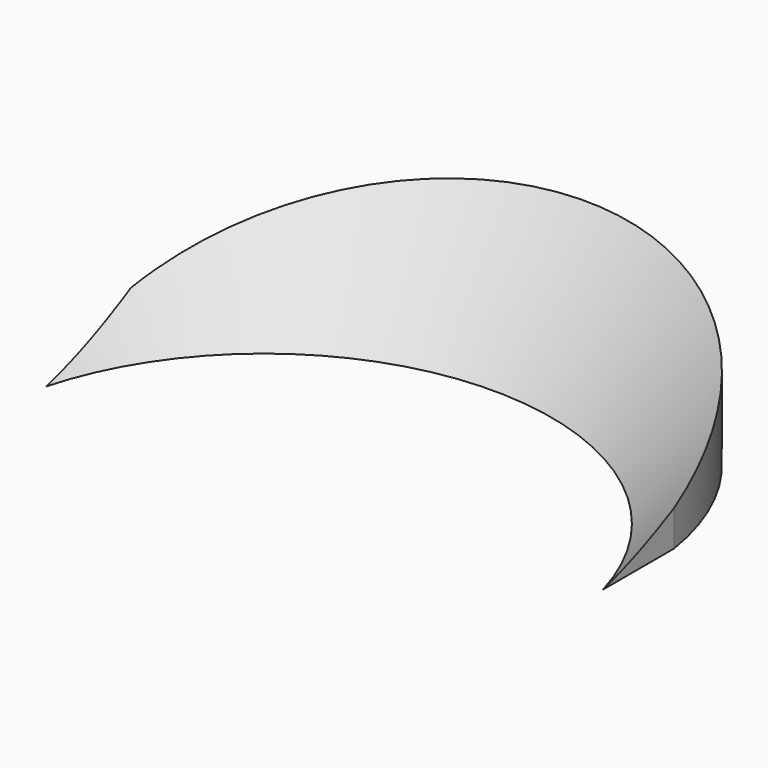
from build123d import *

# Parameters (mm, degrees)
F0_W        = 206.9673240185
F0_H        = 93.9061716199
F1_DEPTH    = 38.1
F3_DEPTH    = 38.1
F4_DEPTH    = 38.1
F5_T4_ANGLE = 333.9674626616
F6_W        = 206.9673240185
F6_H        = 38.1
F8_DEPTH    = 152.4


# Not quite as in the source:
# - a fillet or chamfer that OpenCascade refuses, or shapes differently, is made with other operations: its cross-section is extruded or revolved along the edge and cut away or added


with BuildPart() as f1:
    # F0 (on Top) → F1 (new body)
    with BuildSketch(Plane.XY):
        with Locations((-103.4836620092, 46.9530858099)):
            Rectangle(F0_W, F0_H)
    extrude(amount=F1_DEPTH)

    # F2 (on face) → F3 (join)
    with BuildSketch(Plane.XY.offset(38.1)):
        with BuildLine():
            Line((-38.5484881699, 19.2711967975), (-38.5484881699, 38.0954556167))
            ThreePointArc((-38.5484881699, 38.0954556167), (-95.9617823939, 88.596121937), (-155.8515280485, 41.0585366189))
            Line((-155.8515280485, 41.0585366189), (-155.8515280485, 19.9683923274))
            ThreePointArc((-155.8515280485, 19.9683923274), (-96.8534760925, 77.9237526804), (-38.5484881699, 19.2711967975))
        make_face()
    extrude(amount=F3_DEPTH)

    # F2 (on face) → F4 (join)
    with BuildSketch(Plane.XY.offset(38.1)):
        with BuildLine():
            ThreePointArc((-155.8515280485, 18.5740012676), (-97.4655811383, 63.6052200178), (-38.5484881699, 19.2711967975))
            ThreePointArc((-38.5484881699, 19.2711967975), (-96.8534760925, 77.9237526804), (-155.8515280485, 19.9683923274))
            Line((-155.8515280485, 19.9683923274), (-155.8515280485, 18.5740012676))
        make_face()
    extrude(amount=F4_DEPTH)

    # F5: chamfer of 38.1 on 1 edges, made by hand


with BuildPart() as f5_tool2:
    # F5_s3 → F5_t4 (revolve)
    with BuildSketch(Plane(origin=(-93.0214210663, 20.9218871248, 0), x_dir=(0, 0, 1), z_dir=(0.9756275706, -0.2194330045, 0))):
        Polygon((38.1, 79.4412595984), (76.2, 117.5412595984), (76.2, 79.4412595984), align=None)
    revolve(axis=Axis((-97.1040055743, 2.7701874098, 76.2), (0, 0, -1)), revolution_arc=F5_T4_ANGLE)

    split(bisect_by=Plane.XY.offset(38.1), keep=Keep.TOP)


with BuildPart() as f1_1:
    add(f1.part)

    # F5_t1: cut F5_tool2
    add(f5_tool2.part, mode=Mode.SUBTRACT)

    # F6 (on face) → F8 (cut)
    with BuildSketch(Plane.XZ):
        with Locations((-103.4836620092, 19.05)):
            Rectangle(F6_W, F6_H)
    extrude(amount=-F8_DEPTH, mode=Mode.SUBTRACT)


solid = f1_1.part
